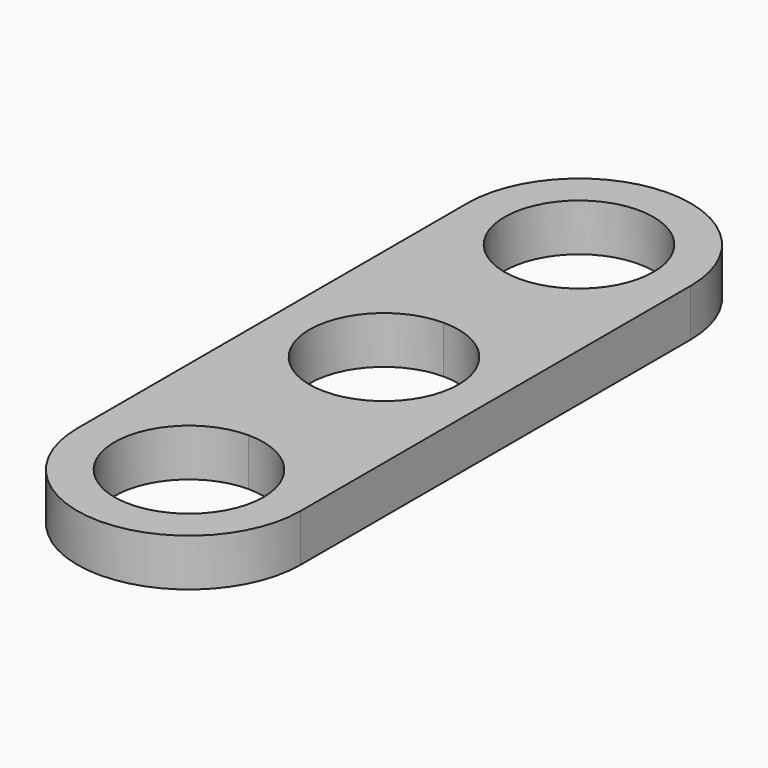
from build123d import *

# Parameters (mm, degrees)
F1_DEPTH = 7


# Not quite as in the source:
# - a feature names something its author has since deleted; it is built from what else it names


with BuildPart() as f1:
    # F0 (on Top) → F1 (new body)
    with BuildSketch(Plane.XY):
        with BuildLine():
            ThreePointArc((0, 11), (7.7781745931, 7.7781745931), (11, 0))
            ThreePointArc((11, 0), (7.7781745931, -7.7781745931), (0, -11))
            Line((0, -11), (0, -16.5))
            ThreePointArc((0, -16.5), (11.6672618896, -11.6672618896), (16.5, 0))
            ThreePointArc((16.5, 0), (11.6672618896, 11.6672618896), (0, 16.5))
            Line((0, 16.5), (0, 11))
        make_face()
        with BuildLine():
            ThreePointArc((0, -11), (-11, 0), (0, 11))
            Line((0, 11), (0, 16.5))
            ThreePointArc((0, 16.5), (-11.6672618896, 11.6672618896), (-16.5, 0))
            ThreePointArc((-16.5, 0), (-11.6672618896, -11.6672618896), (0, -16.5))
            Line((0, -16.5), (0, -11))
        make_face()
        with BuildLine():
            Line((0, 19.5), (0, 16.5))
            ThreePointArc((0, 16.5), (11.6672618896, 11.6672618896), (16.5, 0))
            Line((16.5, 0), (16.5, 36))
            ThreePointArc((16.5, 36), (11.6672618896, 24.3327381104), (0, 19.5))
        make_face()
        with BuildLine():
            ThreePointArc((-16.5, 0), (-11.6672618896, 11.6672618896), (0, 16.5))
            Line((0, 16.5), (0, 19.5))
            ThreePointArc((0, 19.5), (-11.6672618896, 24.3327381104), (-16.5, 36))
            Line((-16.5, 36), (-16.5, 0))
        make_face()
        with BuildLine():
            Line((0, -19.5), (0, -16.5))
            ThreePointArc((0, -16.5), (-11.6672618896, -11.6672618896), (-16.5, 0))
            Line((-16.5, 0), (-16.5, -36))
            ThreePointArc((-16.5, -36), (-11.6672618896, -24.3327381104), (0, -19.5))
        make_face()
        with BuildLine():
            ThreePointArc((16.5, 0), (11.6672618896, -11.6672618896), (0, -16.5))
            Line((0, -16.5), (0, -19.5))
            ThreePointArc((0, -19.5), (11.6672618896, -24.3327381104), (16.5, -36))
            Line((16.5, -36), (16.5, 0))
        make_face()
        with BuildLine():
            ThreePointArc((-16.5, 36), (-11.6672618896, 24.3327381104), (0, 19.5))
            ThreePointArc((0, 19.5), (11.6672618896, 24.3327381104), (16.5, 36))
            ThreePointArc((16.5, 36), (0, 52.5), (-16.5, 36))
        make_face()
        with BuildLine():
            ThreePointArc((11, 36), (7.7781745931, 28.2218254069), (0, 25))
            ThreePointArc((0, 25), (-7.7781745931, 43.7781745931), (11, 36))
        make_face(mode=Mode.SUBTRACT)
        with BuildLine():
            ThreePointArc((16.5, -36), (11.6672618896, -24.3327381104), (0, -19.5))
            ThreePointArc((0, -19.5), (-11.6672618896, -24.3327381104), (-16.5, -36))
            ThreePointArc((-16.5, -36), (0, -52.5), (16.5, -36))
        make_face()
        with BuildLine():
            ThreePointArc((11, -36), (-7.7781745931, -43.7781745931), (0, -25))
            ThreePointArc((0, -25), (7.7781745931, -28.2218254069), (11, -36))
        make_face(mode=Mode.SUBTRACT)
    extrude(amount=F1_DEPTH)


solid = f1.part
